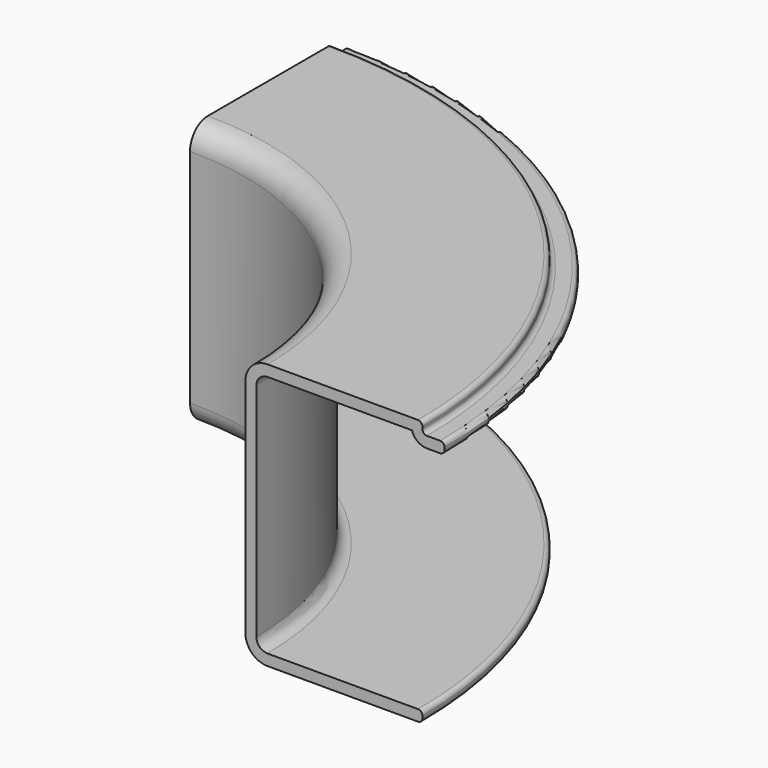
from build123d import *

# Parameters (mm, degrees)
F1_ANGLE = 90


# Not quite as in the source:
# - ends of sketch curves that miss each other by under 0.0002 mm in the source are joined


with BuildPart() as f1:
    # F0 (on Front) → F1 (revolve)
    with BuildSketch(Plane.XZ):
        with BuildLine():
            Line((158.75, 139.7), (158.75, 12.7))
            ThreePointArc((158.75, 12.7), (162.4697438789, 3.7197438789), (171.45, 0))
            Line((171.45, 0), (257.81, 0))
            ThreePointArc((257.81, 0), (259.6060512242, 0.7439487758), (260.35, 2.54))
            Line((260.35, 2.54), (260.35, 3.8099999233))
            ThreePointArc((260.35, 3.8099999233), (259.6060512242, 5.6060511475), (257.81, 6.3499999233))
            Line((257.81, 6.3499999233), (171.45, 6.3499999233))
            ThreePointArc((171.45, 6.3499999233), (166.9598694704, 8.2098694704), (165.0999965083, 12.7))
            Line((165.0999965083, 12.7), (165.1, 139.7))
            ThreePointArc((165.1, 139.7), (166.9598719395, 144.1901280605), (171.45, 146.05))
            Line((171.45, 146.05), (254.3705810057, 146.05))
            ThreePointArc((254.3705810057, 146.05), (257.5772088315, 141.4621426782), (262.89, 139.7))
            Line((262.89, 139.7), (270.51, 139.7))
            ThreePointArc((270.51, 139.7), (272.3060512242, 140.4439487758), (273.05, 142.24))
            Line((273.05, 142.24), (273.05, 143.51))
            ThreePointArc((273.05, 143.51), (272.3060512242, 145.3060512242), (270.51, 146.05))
            Line((270.51, 146.05), (262.89, 146.05))
            ThreePointArc((262.89, 146.05), (261.0939487758, 146.7939487758), (260.35, 148.59))
            Line((260.35, 148.59), (260.35, 149.86))
            ThreePointArc((260.35, 149.86), (259.6060512242, 151.6560512242), (257.81, 152.4))
            Line((257.81, 152.4), (171.45, 152.4))
            ThreePointArc((171.45, 152.4), (162.4697438789, 148.6802561211), (158.75, 139.7))
        make_face()
    revolve(axis=Axis((0, 0, 68.397693336), (0, 0, 1)), revolution_arc=F1_ANGLE)


solid = f1.part
